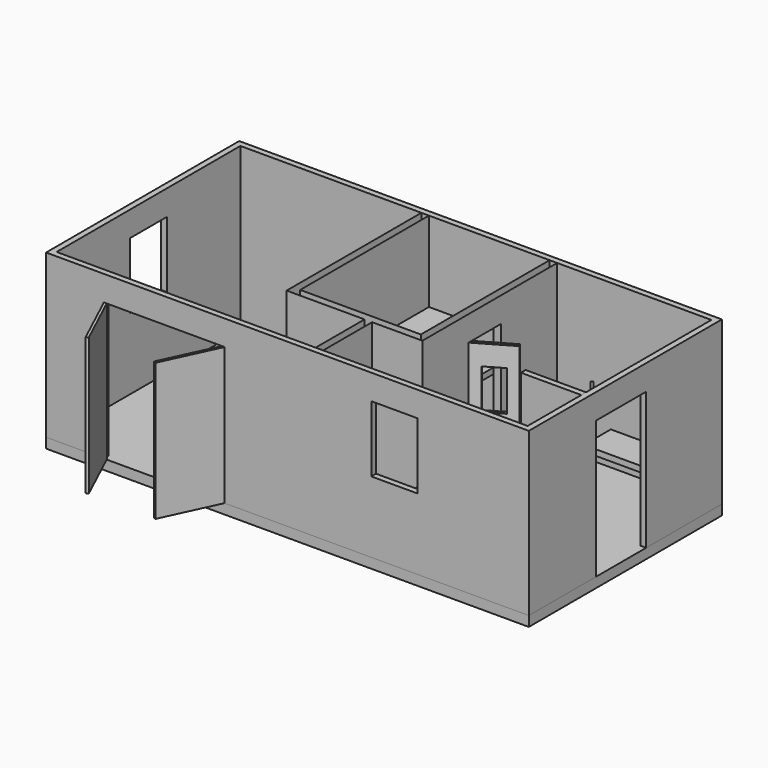
from build123d import *

# Parameters (mm, degrees)
F0_W           = 7315.2
F0_H           = 3657.6
F1_DEPTH       = 152.4
F2_W           = 7315.2
F2_H           = 3657.6
F2_W_2         = 7137.4
F2_H_2         = 3479.8
F3_DEPTH       = 2463.8
F4_W           = 952.5
F4_H           = 2082.8
F5_DEPTH       = 88.9
F6_W           = 1828.8
F6_H           = 2082.8
F6_W_2         = 698.5
F6_H_2         = 1003.3
F7_DEPTH       = 88.9
F8_W           = 698.5
F8_H           = 1003.3
F9_DEPTH       = 88.9
F10_W          = 114.3
F10_H          = 927.1
F11_DEPTH      = 2463.8
F12_W          = 914.4
F12_H          = 88.9
F13_DEPTH      = 2463.8
F14_W          = 609.6
F14_H          = 2082.8
F15_DEPTH      = 114.3
F16_W          = 609.6
F16_H          = 88.9
F17_DEPTH      = 698.5
F17_DEPTH_BACK = 1739.9
F18_W          = 457.2
F18_H          = 88.9
F19_DEPTH      = 698.5
F19_DEPTH_BACK = 1739.9
F20_W          = 1524
F20_H          = 88.9
F21_DEPTH      = 508
F24_DEPTH      = 2082.8
F26_DEPTH      = 2082.8
F28_DEPTH      = 1676.4
F29_W          = 768.35
F29_H          = 768.35
F30_DEPTH      = 50.8
F31_W          = 1524
F31_H          = 88.9
F32_DEPTH      = 508
F34_DEPTH      = 88.9
F35_W          = 304.8
F35_H          = 609.6
F36_DEPTH      = 50.8
F38_DEPTH      = 50.8
F40_DEPTH      = 25.4
F41_W          = 508
F41_H          = 406.4
F42_DEPTH      = 9.525
F43_W          = 508
F43_H          = 406.4
F43_W_2        = 488.95
F43_H_2        = 387.35
F44_DEPTH      = 406.4
F46_DEPTH      = 12.7
F49_DEPTH      = 2082.8
F50_R          = 304.8
F51_DEPTH      = 914.4
F52_T          = -6.35
F53_W          = 762
F53_H          = 927.1
F54_DEPTH      = 38.1
F55_W          = 393.7
F55_H          = 508
F56_DEPTH      = 114.3


with BuildPart() as f1:
    # F0 (on Top) → F1 (new body)
    with BuildSketch(Plane.XY):
        Rectangle(F0_W, F0_H)
    extrude(amount=F1_DEPTH)


with BuildPart() as f3:
    # F2 (on face) → F3 (new body)
    with BuildSketch(Plane.XY.offset(152.4)):
        Rectangle(F2_W, F2_H)
        Rectangle(F2_W_2, F2_H_2, mode=Mode.SUBTRACT)
    extrude(amount=F3_DEPTH)

    # F4 (on face) → F5 (cut, through all)
    with BuildSketch(Plane.YZ.offset(3657.6)):
        with Locations((-82.55, 1193.8)):
            Rectangle(F4_W, F4_H)
    extrude(amount=-F5_DEPTH, mode=Mode.SUBTRACT)

    # F6 (on face) → F7 (cut, through all)
    with BuildSketch(Plane.XZ.offset(1828.8)):
        with Locations((-1866.9, 1193.8)):
            Rectangle(F6_W, F6_H)
        with Locations((1619.25, 1733.55)):
            Rectangle(F6_W_2, F6_H_2)
    extrude(amount=-F7_DEPTH, mode=Mode.SUBTRACT)

    # F8 (on face) → F9 (cut, through all)
    with BuildSketch(Plane(origin=(-3657.6, 0, 0), x_dir=(0, -1, 0), z_dir=(-1, 0, 0))):
        with Locations((0, 1733.55)):
            Rectangle(F8_W, F8_H)
    extrude(amount=-F9_DEPTH, mode=Mode.SUBTRACT)


with BuildPart() as f11:
    # F10 (on face) → F11 (new body, through all)
    with BuildSketch(Plane.XY.offset(152.4)):
        with Locations((412.75, -1276.35)):
            Rectangle(F10_W, F10_H)
        Polygon((-825.5, -812.8), (355.6, -812.8), (469.9, -812.8), (1231.9, -812.8), (1231.9, 1739.9), (1117.6, 1739.9), (1117.6, -698.5), (-711.2, -698.5), (-711.2, 1739.9), (-825.5, 1739.9), align=None)
    extrude(amount=F11_DEPTH)

    # F14 (on face) → F15 (cut, through all)
    with BuildSketch(Plane.YZ.offset(1231.9)):
        with Locations((368.3, 1193.8)):
            Rectangle(F14_W, F14_H)
    extrude(amount=-F15_DEPTH, mode=Mode.SUBTRACT)

    # F55 (on face) → F56 (cut, through all)
    with BuildSketch(Plane.YZ.offset(1231.9)):
        with Locations((1359.3832832336, 406.4)):
            Rectangle(F55_W, F55_H)
    extrude(amount=-F56_DEPTH, mode=Mode.SUBTRACT)


with BuildPart() as f13:
    # F12 (on face) → F13 (new body, through all)
    with BuildSketch(Plane.XY.offset(152.4)):
        with Locations((3111.5, -679.45)):
            Rectangle(F12_W, F12_H)
    extrude(amount=F13_DEPTH)


with BuildPart() as f17:
    # F16 (on Front) → F17 (new body, two sides)
    with BuildSketch(Plane.XZ) as f17_sk:
        with Locations((-406.4, 1352.55)):
            Rectangle(F16_W, F16_H)
    extrude(amount=F17_DEPTH)
    extrude(f17_sk.sketch, amount=-F17_DEPTH_BACK)


with BuildPart() as f19:
    # F18 (on Front) → F19 (new body, two sides)
    with BuildSketch(Plane.XZ) as f19_sk:
        with Locations((76.2, 895.35)):
            Rectangle(F18_W, F18_H)
    extrude(amount=F19_DEPTH)
    extrude(f19_sk.sketch, amount=-F19_DEPTH_BACK)


with BuildPart() as f21:
    # F20 (on face) → F21 (new body)
    with BuildSketch(Plane.XZ.offset(-1739.9)):
        with Locations((2806.7, 615.95)):
            Rectangle(F20_W, F20_H)
    extrude(amount=F21_DEPTH)


with BuildPart() as f24:
    # F23 (on face) → F24 (new body)
    with BuildSketch(Plane.XY.offset(152.4)):
        Polygon((1734.429086147, 412.2940905122), (1206.5, 107.4940905122), (1231.9, 63.5), (1759.829086147, 368.3), align=None)
    extrude(amount=F24_DEPTH)

    # F35 (on face) → F36 (cut, through all)
    with BuildSketch(Plane(origin=(280.4786934298, -485.803347461, 0), x_dir=(0.8660254038, 0.5, 0), z_dir=(0.5, -0.8660254038, 0))):
        with Locations((1403.406694922, 1625.6)):
            Rectangle(F35_W, F35_H)
    extrude(amount=-F36_DEPTH, mode=Mode.SUBTRACT)


with BuildPart() as f26:
    # F25 (on face) → F26 (new body)
    with BuildSketch(Plane.XY.offset(152.4)):
        Polygon((2977.9257969634, 188.3560018005), (3568.7, -558.8), (3598.586240072, -535.1690318785), (3007.8120370354, 211.986969922), align=None)
    extrude(amount=F26_DEPTH)


with BuildPart() as f28:
    # F27 (on face) → F28 (new body)
    with BuildSketch(Plane.XY.offset(152.4)):
        Polygon((-711.2, -971.55), (-711.2, -1739.9), (57.15, -1739.9), (57.15, -1733.55), (-704.85, -1733.55), (-704.85, -971.55), align=None)
    extrude(amount=F28_DEPTH)

    # F29 (on face) → F30 (join)
    with BuildSketch(Plane.XY.offset(152.4)):
        with Locations((-327.025, -1355.725)):
            Rectangle(F29_W, F29_H)
    extrude(amount=F30_DEPTH)


with BuildPart() as f32:
    # F31 (on face) → F32 (new body)
    with BuildSketch(Plane(origin=(0, -1739.9, 0), x_dir=(-1, 0, 0), z_dir=(0, 1, 0))):
        with Locations((-2806.7, 615.95)):
            Rectangle(F31_W, F31_H)
    extrude(amount=F32_DEPTH)

    # F33 (on face) → F34 (cut, through all)
    with BuildSketch(Plane.XY.offset(660.4)):
        Polygon((2197.1, -1231.9), (2044.7, -1231.9), (2044.7, -1384.3), align=None)
    extrude(amount=-F34_DEPTH, mode=Mode.SUBTRACT)


with BuildPart() as f38:
    # F37 (on face) → F38 (new body)
    with BuildSketch(Plane.XY.offset(152.4)):
        Polygon((508, 977.9), (1117.6, 977.9), (1117.6, 1162.05), (1219.2, 1162.05), (1219.2, 1555.75), (1117.6, 1555.75), (1117.6, 1739.9), (508, 1739.9), align=None)
    extrude(amount=F38_DEPTH)


with BuildPart() as f40:
    # F39 (on face) → F40 (new body)
    with BuildSketch(Plane.XY.offset(152.4)):
        Polygon((1108.0693342209, 1665.9335847944), (1108.0693342209, 1056.3335847944), (1311.2693342209, 1056.3335847944), (1412.8693342209, 1157.9335847944), (1412.8693342209, 1564.3335847944), (1311.2693342209, 1665.9335847944), align=None)
    extrude(amount=F40_DEPTH)


with BuildPart() as f42:
    # F41 (on face) → F42 (new body)
    with BuildSketch(Plane.XY.offset(152.4)):
        with Locations((2629.7176399231, -1536.7)):
            Rectangle(F41_W, F41_H)
    extrude(amount=F42_DEPTH)

    # F43 (on face) → F44 (join)
    with BuildSketch(Plane.XY.offset(161.925)):
        with Locations((2629.7176399231, -1536.7)):
            Rectangle(F43_W, F43_H)
        with Locations((2629.7176399231, -1536.7)):
            Rectangle(F43_W_2, F43_H_2, mode=Mode.SUBTRACT)
    extrude(amount=F44_DEPTH)

    # F45 (on face) → F46 (join)
    with BuildSketch(Plane.XY.offset(568.325)):
        with BuildLine():
            Line((2350.3176399231, -1600.2), (2375.7176399231, -1600.2))
            Line((2375.7176399231, -1600.2), (2375.7176399231, -1473.2))
            Line((2375.7176399231, -1473.2), (2350.3176399231, -1473.2))
            ThreePointArc((2350.3176399231, -1473.2), (2341.337383802, -1476.9197438789), (2337.6176399231, -1485.9))
            Line((2337.6176399231, -1485.9), (2337.6176399231, -1587.5))
            ThreePointArc((2337.6176399231, -1587.5), (2341.337383802, -1596.4802561211), (2350.3176399231, -1600.2))
        make_face()
        with BuildLine():
            Line((2883.7176399231, -1473.2), (2883.7176399231, -1600.2))
            Line((2883.7176399231, -1600.2), (2909.1176399231, -1600.2))
            ThreePointArc((2909.1176399231, -1600.2), (2918.0978960442, -1596.4802561211), (2921.8176399231, -1587.5))
            Line((2921.8176399231, -1587.5), (2921.8176399231, -1485.9))
            ThreePointArc((2921.8176399231, -1485.9), (2918.0978960442, -1476.9197438789), (2909.1176399231, -1473.2))
            Line((2909.1176399231, -1473.2), (2883.7176399231, -1473.2))
        make_face()
    extrude(amount=-F46_DEPTH)


with BuildPart() as f49:
    # F48 (on face) → F49 (new body)
    with BuildSketch(Plane.XY.offset(152.4)):
        Polygon((-2746.7712332818, -1812.6948992887), (-2781.3, -1828.8), (-2394.7775829299, -2657.490401237), (-2360.2488162117, -2641.3853005257), align=None)
    extrude(amount=F49_DEPTH)


with BuildPart() as f49b:
    # F48 (on face) → F49, piece 2 (new body)
    with BuildSketch(Plane.XY.offset(152.4)):
        Polygon((-1339.0224170701, -2657.490401237), (-952.5, -1828.8), (-987.0287667182, -1812.6948992887), (-1373.5511837883, -2641.3853005257), align=None)
    extrude(amount=F49_DEPTH)


with BuildPart() as f51:
    # F50 (on face) → F51 (new body)
    with BuildSketch(Plane.XY.offset(152.4)):
        with Locations((1960.6037139893, -1393.118262291)):
            Circle(F50_R)
    extrude(amount=F51_DEPTH)

    # F52
    f52_openings = [f51.faces().sort_by_distance(p)[0] for p in [
        (1960.603714, -1393.118262, 1066.8),
    ]]
    offset(amount=F52_T, openings=f52_openings)


with BuildPart() as f54:
    # F53 (on face) → F54 (new body)
    with BuildSketch(Plane.XY.offset(152.4)):
        with Locations((850.9, -1276.35)):
            Rectangle(F53_W, F53_H)
    extrude(amount=F54_DEPTH)


solid = Compound([f1.part, f3.part, f11.part, f13.part, f17.part, f19.part, f21.part, f24.part, f26.part, f28.part, f32.part, f38.part, f40.part, f42.part, f49.part, f49b.part, f51.part, f54.part])
